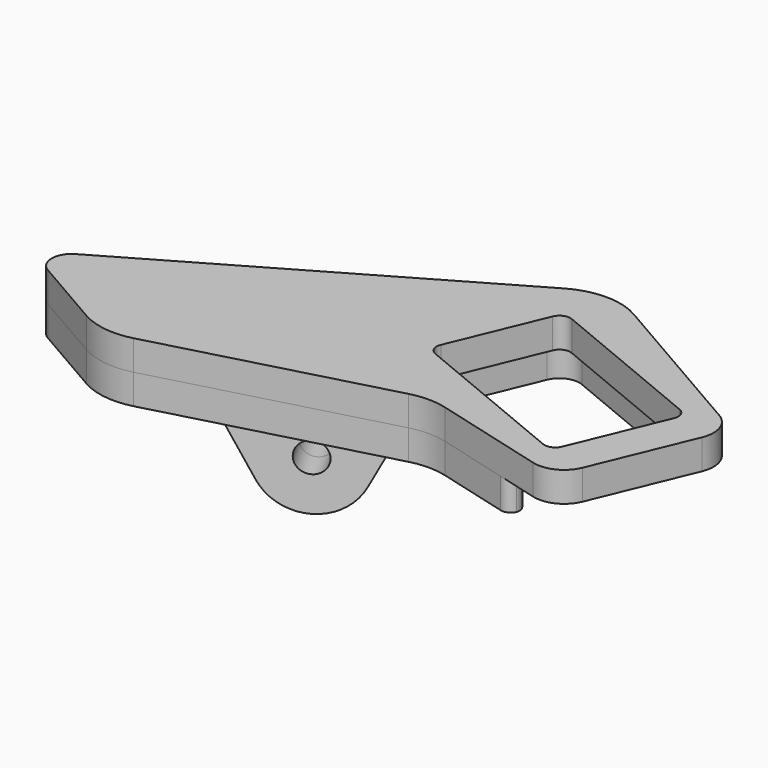
from build123d import *

# Parameters (mm, degrees)
F1_DEPTH     = 3
F3_DEPTH     = 3
F6_R         = 1.5
F6_W         = 10
F6_H         = 3
F7_DEPTH     = 3
F9_OFFSET    = 0.1
F11_DEPTH    = 25
F12_T1_DEPTH = 7.384882315
F12_T3_DEPTH = 8


# Not quite as in the source:
# - a fillet or chamfer that OpenCascade refuses, or shapes differently, is made with other operations: its cross-section is extruded or revolved along the edge and cut away or added


with BuildPart() as f1:
    # F0 (on Top) → F1 (new body)
    with BuildSketch(Plane.XY):
        with BuildLine():
            Line((-3.5, 21.0732848254), (-37, 1.7320508076))
            ThreePointArc((-37, 1.7320508076), (-38, 0), (-37, -1.7320508076))
            Line((-37, -1.7320508076), (-29.8315443489, -5.8707606074))
            ThreePointArc((-29.8315443489, -5.8707606074), (-27.2452276945, -6.7486968105), (-24.5198110332, -6.5700635649))
            Line((-24.5198110332, -6.5700635649), (-1.8117333157, -0.4854524788))
            ThreePointArc((-1.8117333157, -0.4854524788), (0, -0.2469332629), (1.8117333157, -0.4854524788))
            Line((1.8117333157, -0.4854524788), (13.0880962857, -3.5069448302))
            ThreePointArc((13.0880962857, -3.5069448302), (15.1914194917, -3.299785576), (16.6361920186, -1.7572176484))
            Line((16.6361920186, -1.7572176484), (20.725816557, 8.1160093774))
            ThreePointArc((20.725816557, 8.1160093774), (20.794968348, 10.2283780704), (19.4541779595, 11.8621358858))
            Line((19.4541779595, 11.8621358858), (3.5, 21.0732848254))
            ThreePointArc((3.5, 21.0732848254), (0, 22.0111069989), (-3.5, 21.0732848254))
        make_face()
        with BuildLine():
            Line((17.8162192325, 8.9309978447), (13.9893849089, -0.3077974804))
            ThreePointArc((13.9893849089, -0.3077974804), (12.9069927086, -1.3901896807), (11.3762589791, -1.3901896807))
            Line((11.3762589791, -1.3901896807), (-4.7916328398, 5.3067703857))
            ThreePointArc((-4.7916328398, 5.3067703857), (-5.8740250401, 6.389162586), (-5.8740250401, 7.9198963155))
            Line((-5.8740250401, 7.9198963155), (-2.0471907165, 17.1586916406))
            ThreePointArc((-2.0471907165, 17.1586916406), (-0.9647985162, 18.2410838409), (0.5659352133, 18.2410838409))
            Line((0.5659352133, 18.2410838409), (16.7338270322, 11.5441237745))
            ThreePointArc((16.7338270322, 11.5441237745), (17.8162192325, 10.4617315742), (17.8162192325, 8.9309978447))
        make_face(mode=Mode.SUBTRACT)
    extrude(amount=F1_DEPTH)


with BuildPart() as f3:
    # F2 (on face) → F3 (new body)
    with BuildSketch(Plane.XY.offset(3)):
        with BuildLine():
            Line((1.8117333157, -0.4854524788), (13.0880962857, -3.5069448302))
            ThreePointArc((13.0880962857, -3.5069448302), (15.1914194917, -3.299785576), (16.6361920186, -1.7572176484))
            Line((16.6361920186, -1.7572176484), (20.725816557, 8.1160093774))
            ThreePointArc((20.725816557, 8.1160093774), (20.794968348, 10.2283780704), (19.4541779595, 11.8621358858))
            Line((19.4541779595, 11.8621358858), (3.5, 21.0732848254))
            ThreePointArc((3.5, 21.0732848254), (0, 22.0111069989), (-3.5, 21.0732848254))
            Line((-3.5, 21.0732848254), (-37, 1.7320508076))
            ThreePointArc((-37, 1.7320508076), (-38, 0), (-37, -1.7320508076))
            Line((-37, -1.7320508076), (-29.8315443489, -5.8707606074))
            ThreePointArc((-29.8315443489, -5.8707606074), (-27.2452276945, -6.7486968105), (-24.5198110332, -6.5700635649))
            Line((-24.5198110332, -6.5700635649), (-1.8117333157, -0.4854524788))
            ThreePointArc((-1.8117333157, -0.4854524788), (0, -0.2469332629), (1.8117333157, -0.4854524788))
        make_face()
        with BuildLine():
            ThreePointArc((-4.4472177507, 6.138261965), (-5.0425334609, 6.7335776751), (-5.0425334609, 7.5754812264))
            Line((-5.0425334609, 7.5754812264), (-1.2156991372, 16.8142765515))
            ThreePointArc((-1.2156991372, 16.8142765515), (-0.620383427, 17.4095922616), (0.2215201242, 17.4095922616))
            Line((0.2215201242, 17.4095922616), (16.3894119431, 10.7126321952))
            ThreePointArc((16.3894119431, 10.7126321952), (16.9847276533, 10.1173164851), (16.9847276533, 9.2754129339))
            Line((16.9847276533, 9.2754129339), (13.1578933296, 0.0366176088))
            ThreePointArc((13.1578933296, 0.0366176088), (12.5625776195, -0.5586981014), (11.7206740683, -0.5586981014))
            Line((11.7206740683, -0.5586981014), (-4.4472177507, 6.138261965))
        make_face(mode=Mode.SUBTRACT)
    extrude(amount=F3_DEPTH)


with BuildPart() as f7:
    # F6 (on offset) → F7 (new body)
    with BuildSketch(Plane(origin=(-8.75, 15.1554445662, 0), x_dir=(-0.8660254038, -0.5, 0), z_dir=(-0.5, 0.8660254038, 0))):
        with BuildLine():
            ThreePointArc((15.6119687021, -8.3087430662), (16.0336248853, -7.1884294616), (16.1769145362, -6))
            ThreePointArc((16.1769145362, -6), (9.9884850746, -1.1432896509), (6.7418603703, -8.3087430662))
            ThreePointArc((6.7418603703, -8.3087430662), (11.1769145362, -11), (15.6119687021, -8.3087430662))
        make_face()
        with Locations((11.1769145362, -6)):
            Circle(F6_R, mode=Mode.SUBTRACT)
        with BuildLine():
            ThreePointArc((6.7418603703, -8.3087430662), (9.9884850746, -1.1432896509), (16.1769145362, -6))
            ThreePointArc((16.1769145362, -6), (16.0336248853, -7.1884294616), (15.6119687021, -8.3087430662))
            Line((15.6119687021, -8.3087430662), (19.9372265739, 0))
            Line((19.9372265739, 0), (16.1769145362, 0))
            Line((16.1769145362, 0), (6.1769145362, 0))
            Line((6.1769145362, 0), (2.4166024986, 0))
            Line((2.4166024986, 0), (6.7418603703, -8.3087430662))
        make_face()
        with Locations((11.1769145362, 1.5)):
            Rectangle(F6_W, F6_H)
    extrude(amount=-F7_DEPTH)


with BuildPart() as f8_1:
    # F8: copy of F7
    add(f7.part.moved(Location((1.5, -2.5980762114, 0))))


with BuildPart() as f1_1:
    add(f1.part)

    # F9: cut F8_1, F7, each made larger all round first
    f9_tool = offset(f8_1.part, amount=F9_OFFSET, kind=Kind.INTERSECTION, mode=Mode.PRIVATE)
    add(f9_tool, mode=Mode.SUBTRACT)
    f9_tool1 = offset(f7.part, amount=F9_OFFSET, kind=Kind.INTERSECTION, mode=Mode.PRIVATE)
    add(f9_tool1, mode=Mode.SUBTRACT)

    # F10 (on face) → F11 (cut)
    with BuildSketch(Plane(origin=(0, 0, 0), x_dir=(1, 0, 0), z_dir=(0, 0, -1))):
        Polygon((8.0851493308, 6.7225052992), (10.4523794466, 1.0075062483), (16.4916398288, -13.5725580731), (23.6928509238, -13.6364949582), (14.2091623748, 9.2591545582), align=None)
    extrude(amount=-F11_DEPTH, mode=Mode.SUBTRACT)

    # F12: fillet of radius 1 on 4 edges, made by hand

    # F12_s2 → F12_t1 (cut)
    with BuildSketch(Plane.XY.offset(-2.1924411575)):
        with BuildLine():
            ThreePointArc((8.936720142, -2.394586945), (9.6378278773, -2.3255338603), (10.1194187196, -1.8113445511))
            Line((10.1194187196, -1.8113445511), (9.7838143567, -2.6215651558))
            Line((9.7838143567, -2.6215651558), (8.936720142, -2.394586945))
        make_face()
        with BuildLine():
            ThreePointArc((15.7321559333, 14.0110463045), (16.1790860628, 13.4664603661), (16.1560354658, 12.7623374684))
            Line((16.1560354658, 12.7623374684), (16.4916398288, 13.5725580731))
            Line((16.4916398288, 13.5725580731), (15.7321559333, 14.0110463045))
        make_face()
    extrude(amount=F12_T1_DEPTH, mode=Mode.SUBTRACT)

    # F12_s4 → F12_t3 (cut)
    with BuildSketch(Plane.XY.offset(-2.5)):
        with BuildLine():
            ThreePointArc((10.0696960143, -1.9313857808), (10.0696960143, -1.1660189161), (9.5284999141, -0.6248228159))
            Line((9.5284999141, -0.6248228159), (10.4523794466, -1.0075062483))
            Line((10.4523794466, -1.0075062483), (10.0696960143, -1.9313857808))
        make_face()
        with BuildLine():
            ThreePointArc((16.1926309321, 12.8506867394), (15.6514348319, 12.3094906392), (14.8860679672, 12.3094906392))
            Line((14.8860679672, 12.3094906392), (15.8099474997, 11.9268072069))
            Line((15.8099474997, 11.9268072069), (16.1926309321, 12.8506867394))
        make_face()
    extrude(amount=F12_T3_DEPTH, mode=Mode.SUBTRACT)


with BuildPart() as f3_1:
    add(f3.part)

    # F9: cut F8_1, F7, each made larger all round first
    f9_tool = offset(f8_1.part, amount=F9_OFFSET, kind=Kind.INTERSECTION, mode=Mode.PRIVATE)
    add(f9_tool, mode=Mode.SUBTRACT)
    f9_tool1 = offset(f7.part, amount=F9_OFFSET, kind=Kind.INTERSECTION, mode=Mode.PRIVATE)
    add(f9_tool1, mode=Mode.SUBTRACT)


solid = Compound([f7.part, f8_1.part, f1_1.part, f3_1.part])
